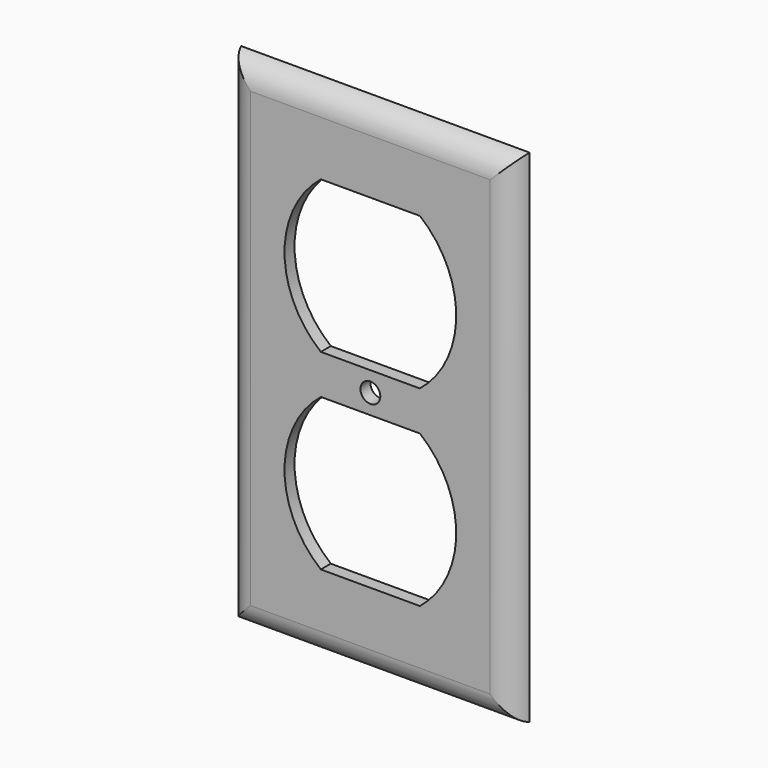
from build123d import *

# Parameters (mm, degrees)
F0_W        = 58.42
F0_H        = 101.6
F1_DEPTH    = 3.81
F2_T1_DEPTH = 126.1934442484
F2_T3_DEPTH = 83.0134442484
F4_T        = -2.54
F3_R        = 2.0082426315
F5_DEPTH    = 25.4


# Not quite as in the source:
# - a fillet or chamfer that OpenCascade refuses, or shapes differently, is made with other operations: its cross-section is extruded or revolved along the edge and cut away or added


with BuildPart() as f1:
    # F0 (on Front) → F1 (new body)
    with BuildSketch(Plane.XZ):
        Rectangle(F0_W, F0_H)
    extrude(amount=F1_DEPTH)

    # F2: fillet of radius 5.08 on 4 edges, made by hand

    # F2_s2 → F2_t1 (cut)
    with BuildSketch(Plane.XY.offset(-63.0967221242)):
        with BuildLine():
            ThreePointArc((-29.21, 0), (-27.4021631237, -2.7460926284), (-24.2913111503, -3.81))
            Line((-24.2913111503, -3.81), (-24.2913111503, -3.9116))
            Line((-24.2913111503, -3.9116), (-29.21, -3.9116))
            Line((-29.21, -3.9116), (-29.3116, -3.81))
            ThreePointArc((-29.3116, -3.81), (-29.3116, -1.905), (-29.308373777, -0.0254))
            Line((-29.308373777, -0.0254), (-29.21, 0))
        make_face()
        with BuildLine():
            ThreePointArc((29.21, 0), (27.4021631237, -2.7460926284), (24.2913111503, -3.81))
            Line((24.2913111503, -3.81), (24.2913111503, -3.9116))
            Line((24.2913111503, -3.9116), (29.21, -3.9116))
            Line((29.21, -3.9116), (29.3116, -3.81))
            ThreePointArc((29.3116, -3.81), (29.3116, -1.905), (29.308373777, -0.0254))
            Line((29.308373777, -0.0254), (29.21, 0))
        make_face()
    extrude(amount=F2_T1_DEPTH, mode=Mode.SUBTRACT)

    # F2_s4 → F2_t3 (cut)
    with BuildSketch(Plane.YZ.offset(-41.5067221242)):
        with BuildLine():
            ThreePointArc((0, 50.8), (-2.7460926284, 48.9921631237), (-3.81, 45.8813111503))
            Line((-3.81, 45.8813111503), (-3.9116, 45.8813111503))
            Line((-3.9116, 45.8813111503), (-3.9116, 50.8))
            Line((-3.9116, 50.8), (-3.81, 50.9016))
            ThreePointArc((-3.81, 50.9016), (-1.905, 50.9016), (-0.0254, 50.898373777))
            Line((-0.0254, 50.898373777), (0, 50.8))
        make_face()
        with BuildLine():
            ThreePointArc((0, -50.8), (-2.7460926284, -48.9921631237), (-3.81, -45.8813111503))
            Line((-3.81, -45.8813111503), (-3.9116, -45.8813111503))
            Line((-3.9116, -45.8813111503), (-3.9116, -50.8))
            Line((-3.9116, -50.8), (-3.81, -50.9016))
            ThreePointArc((-3.81, -50.9016), (-1.905, -50.9016), (-0.0254, -50.898373777))
            Line((-0.0254, -50.898373777), (0, -50.8))
        make_face()
    extrude(amount=F2_T3_DEPTH, mode=Mode.SUBTRACT)

    # F4
    f4_openings = [f1.faces().sort_by_distance(p)[0] for p in [
        (0, 0, 0),
    ]]
    offset(amount=F4_T, openings=f4_openings)

    # F3 (on face) → F5 (cut)
    with BuildSketch(Plane(origin=(0, 0, 0), x_dir=(-1, 0, 0), z_dir=(0, 1, 0))):
        with BuildLine():
            Line((10.0412131573, 34.8095389452), (-10.0412131573, 34.8095389452))
            ThreePointArc((-10.0412131573, 34.8095389452), (-17.399, 19.413012104), (-10.0412131573, 4.0164852629))
            Line((-10.0412131573, 4.0164852629), (10.0412131573, 4.0164852629))
            ThreePointArc((10.0412131573, 4.0164852629), (17.399, 19.413012104), (10.0412131573, 34.8095389452))
        make_face()
        with BuildLine():
            Line((10.0412131573, -4.0164852629), (-10.0412131573, -4.0164852629))
            ThreePointArc((-10.0412131573, -4.0164852629), (-17.399, -19.413012104), (-10.0412131573, -34.8095389452))
            Line((-10.0412131573, -34.8095389452), (10.0412131573, -34.8095389452))
            ThreePointArc((10.0412131573, -34.8095389452), (17.399, -19.413012104), (10.0412131573, -4.0164852629))
        make_face()
        Circle(F3_R)
    extrude(amount=-F5_DEPTH, mode=Mode.SUBTRACT)


solid = f1.part
